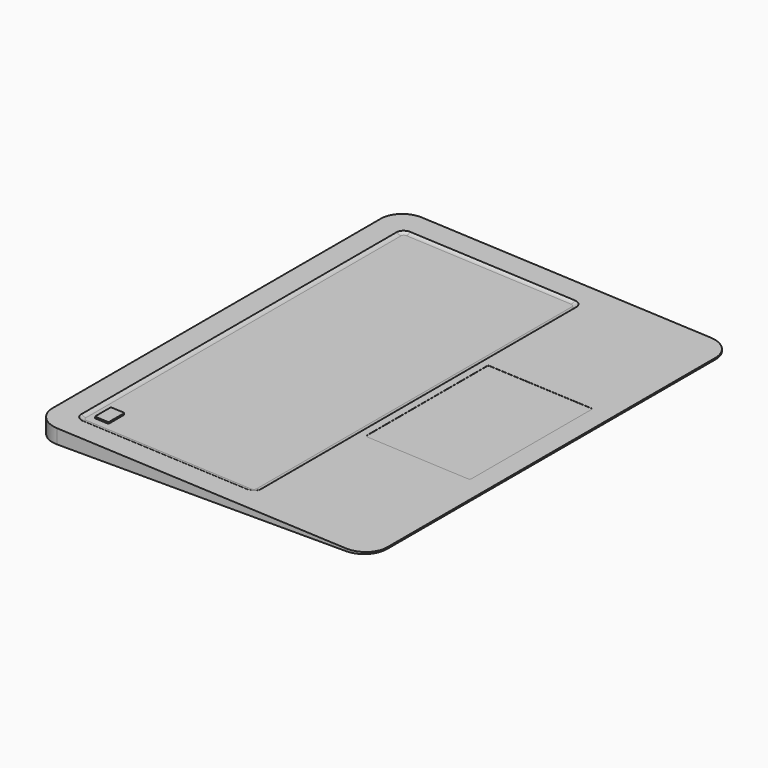
from build123d import *

# Parameters (mm, degrees)
F1_DEPTH     = 300
F2_R         = 15
F4_DEPTH     = 1
F5_T1_DEPTH  = 108.3513065438
F5_T3_DEPTH  = 259.0557519346
F5_T5_DEPTH  = 108.3513065438
F5_T8_ANGLE  = 90
F5_T10_ANGLE = 90
F5_T12_ANGLE = 90
F5_T14_ANGLE = 90
F7_DEPTH     = 0.1
F9_DEPTH     = 1


# Not quite as in the source:
# - a fillet or chamfer that OpenCascade refuses, or shapes differently, is made with other operations: its cross-section is extruded or revolved along the edge and cut away or added


with BuildPart() as f1:
    # F0 (on Front) → F1 (new body)
    with BuildSketch(Plane.XZ):
        Polygon((-88.9504104853, 0), (131.0495895147, 0), (131.0495895147, 1), (-88.9504104853, 10), align=None)
    extrude(amount=F1_DEPTH)

    # F2
    f2_edges = [f1.edges().sort_by_distance(p)[0] for p in [
        (-88.95041, -300, 5),
        (131.04959, -300, 0.5),
        (131.04959, 0, 0.5),
        (-88.95041, 0, 5),
    ]]
    fillet(f2_edges, radius=F2_R)

    # F3 (on face) → F4 (cut)
    with BuildSketch(Plane(origin=(0.2597928415, 0, 6.3504916821), x_dir=(0.999164272, 0, -0.040874902), z_dir=(0.040874902, 0, 0.999164272))):
        with BuildLine():
            ThreePointArc((-74.2722747486, -280), (-72.8078086545, -283.5355339059), (-69.2722747486, -285))
            Line((-69.2722747486, -285), (39.0790317953, -285))
            ThreePointArc((39.0790317953, -285), (42.6145657012, -283.5355339059), (44.0790317953, -280))
            Line((44.0790317953, -280), (44.0790317953, -20.9442480654))
            ThreePointArc((44.0790317953, -20.9442480654), (42.6145657012, -17.4087141594), (39.0790317953, -15.9442480654))
            Line((39.0790317953, -15.9442480654), (-69.2722747486, -15.9442480654))
            ThreePointArc((-69.2722747486, -15.9442480654), (-72.8078086545, -17.4087141594), (-74.2722747486, -20.9442480654))
            Line((-74.2722747486, -20.9442480654), (-74.2722747486, -280))
        make_face()
    extrude(amount=-F4_DEPTH, mode=Mode.SUBTRACT)

    # F5: fillet of radius 5 on 8 edges, made by hand

    # F5_s2 → F5_t1 (join)
    with BuildSketch(Plane(origin=(-69.214381967, 0, 2.8314974441), x_dir=(0, 1, 0), z_dir=(0.999164272, 0, -0.040874902))):
        with BuildLine():
            ThreePointArc((-285, 6.3558034051), (-283.5811388301, 5.6123869149), (-282, 5.3558034051))
            Line((-282, 5.3558034051), (-285, 5.3558034051))
            Line((-285, 5.3558034051), (-285, 6.3558034051))
        make_face()
    extrude(amount=F5_T1_DEPTH)

    # F5_s4 → F5_t3 (join)
    with BuildSketch(Plane.XZ.offset(20.9442480654)):
        with BuildLine():
            ThreePointArc((44.3019865544, 4.5487655756), (42.8539240904, 3.8639661907), (41.2636188365, 3.6722260098))
            Line((41.2636188365, 3.6722260098), (44.2611116524, 3.5496013037))
            Line((44.2611116524, 3.5496013037), (44.3019865544, 4.5487655756))
        make_face()
        with BuildLine():
            ThreePointArc((-73.9504104853, 9.3863636364), (-72.5631221736, 8.5855726288), (-70.9937925714, 8.2645746583))
            Line((-70.9937925714, 8.2645746583), (-73.9912853873, 8.3871993644))
            Line((-73.9912853873, 8.3871993644), (-73.9504104853, 9.3863636364))
        make_face()
    extrude(amount=F5_T3_DEPTH)

    # F5_s6 → F5_t5 (join)
    with BuildSketch(Plane(origin=(39.0463723531, 0, -1.5973515963), x_dir=(0, 1, 0), z_dir=(-0.999164272, 0, 0.040874902))):
        with BuildLine():
            ThreePointArc((-15.9442480654, -6.3558034051), (-17.3631092353, -5.6123869149), (-18.9442480654, -5.3558034051))
            Line((-18.9442480654, -5.3558034051), (-15.9442480654, -5.3558034051))
            Line((-15.9442480654, -5.3558034051), (-15.9442480654, -6.3558034051))
        make_face()
    extrude(amount=F5_T5_DEPTH)

    # F5_s7 → F5_t8 (revolve)
    with BuildSketch(Plane.XZ.offset(280)):
        with BuildLine():
            ThreePointArc((-73.9504104853, 9.3863636364), (-72.5631221736, 8.5855726288), (-70.9937925714, 8.2645746583))
            Line((-70.9937925714, 8.2645746583), (-73.9912853873, 8.3871993644))
            Line((-73.9912853873, 8.3871993644), (-73.9504104853, 9.3863636364))
        make_face()
    revolve(axis=Axis((-68.9954640274, -280, 8.1828248542), (0.040874902, 0, 0.999164272)), revolution_arc=F5_T8_ANGLE)

    # F5_s9 → F5_t10 (revolve)
    with BuildSketch(Plane(origin=(39.046372353, 0, -1.5973515963), x_dir=(0, 1, 0), z_dir=(-0.999164272, 0, 0.040874902))):
        with BuildLine():
            ThreePointArc((-285, -6.3558034051), (-283.5811388301, -5.6123869149), (-282, -5.3558034051))
            Line((-282, -5.3558034051), (-285, -5.3558034051))
            Line((-285, -5.3558034051), (-285, -6.3558034051))
        make_face()
    revolve(axis=Axis((39.2652902926, -280, 3.7539758139), (0.040874902, 0, 0.999164272)), revolution_arc=F5_T10_ANGLE)

    # F5_s11 → F5_t12 (revolve)
    with BuildSketch(Plane.XZ.offset(20.9442480654)):
        with BuildLine():
            ThreePointArc((44.3019865544, 4.5487655756), (42.8539240904, 3.8639661907), (41.2636188365, 3.6722260098))
            Line((41.2636188365, 3.6722260098), (44.2611116524, 3.5496013037))
            Line((44.2611116524, 3.5496013037), (44.3019865544, 4.5487655756))
        make_face()
    revolve(axis=Axis((39.2652902926, -20.9442480654, 3.7539758139), (0.040874902, 0, 0.999164272)), revolution_arc=F5_T12_ANGLE)

    # F5_s13 → F5_t14 (revolve)
    with BuildSketch(Plane(origin=(-69.214381967, 0, 2.8314974441), x_dir=(0, 1, 0), z_dir=(0.999164272, 0, -0.040874902))):
        with BuildLine():
            ThreePointArc((-15.9442480654, 6.3558034051), (-17.3631092353, 5.6123869149), (-18.9442480654, 5.3558034051))
            Line((-18.9442480654, 5.3558034051), (-15.9442480654, 5.3558034051))
            Line((-15.9442480654, 5.3558034051), (-15.9442480654, 6.3558034051))
        make_face()
    revolve(axis=Axis((-68.9954640274, -20.9442480654, 8.1828248542), (0.040874902, 0, 0.999164272)), revolution_arc=F5_T14_ANGLE)

    # F6 (on face) → F7 (cut)
    with BuildSketch(Plane(origin=(0.2597928415, 0, 6.3504916821), x_dir=(0.999164272, 0, -0.040874902), z_dir=(0.040874902, 0, 0.999164272))):
        with BuildLine():
            ThreePointArc((117.753483355, -100.5515882969), (117.4605901362, -99.8444815157), (116.753483355, -99.5515882969))
            Line((116.753483355, -99.5515882969), (49.977278173, -99.5515882969))
            ThreePointArc((49.977278173, -99.5515882969), (49.2701713918, -99.8444815157), (48.977278173, -100.5515882969))
            Line((48.977278173, -100.5515882969), (48.977278173, -199.4484117031))
            ThreePointArc((48.977278173, -199.4484117031), (49.2701713918, -200.1555184843), (49.977278173, -200.4484117031))
            Line((49.977278173, -200.4484117031), (116.753483355, -200.4484117031))
            ThreePointArc((116.753483355, -200.4484117031), (117.4605901362, -200.1555184843), (117.753483355, -199.4484117031))
            Line((117.753483355, -199.4484117031), (117.753483355, -100.5515882969))
        make_face()
    extrude(amount=-F7_DEPTH, mode=Mode.SUBTRACT)

    # F8 (on face) → F9 (join)
    with BuildSketch(Plane(origin=(0.2189179395, 0, 5.3513274101), x_dir=(0.999164272, 0, -0.040874902), z_dir=(0.040874902, 0, 0.999164272))):
        with BuildLine():
            ThreePointArc((-67.5527229905, -276.7879536152), (-67.4062763811, -277.1415070058), (-67.0527229905, -277.2879536152))
            Line((-67.0527229905, -277.2879536152), (-59.0665953457, -277.2879536152))
            ThreePointArc((-59.0665953457, -277.2879536152), (-58.7130419551, -277.1415070058), (-58.5665953457, -276.7879536152))
            Line((-58.5665953457, -276.7879536152), (-58.5665953457, -264.596647501))
            ThreePointArc((-58.5665953457, -264.596647501), (-58.7130419551, -264.2430941104), (-59.0665953457, -264.096647501))
            Line((-59.0665953457, -264.096647501), (-67.0527229905, -264.096647501))
            ThreePointArc((-67.0527229905, -264.096647501), (-67.4062763811, -264.2430941104), (-67.5527229905, -264.596647501))
            Line((-67.5527229905, -264.596647501), (-67.5527229905, -276.7879536152))
        make_face()
    extrude(amount=F9_DEPTH)


solid = f1.part
